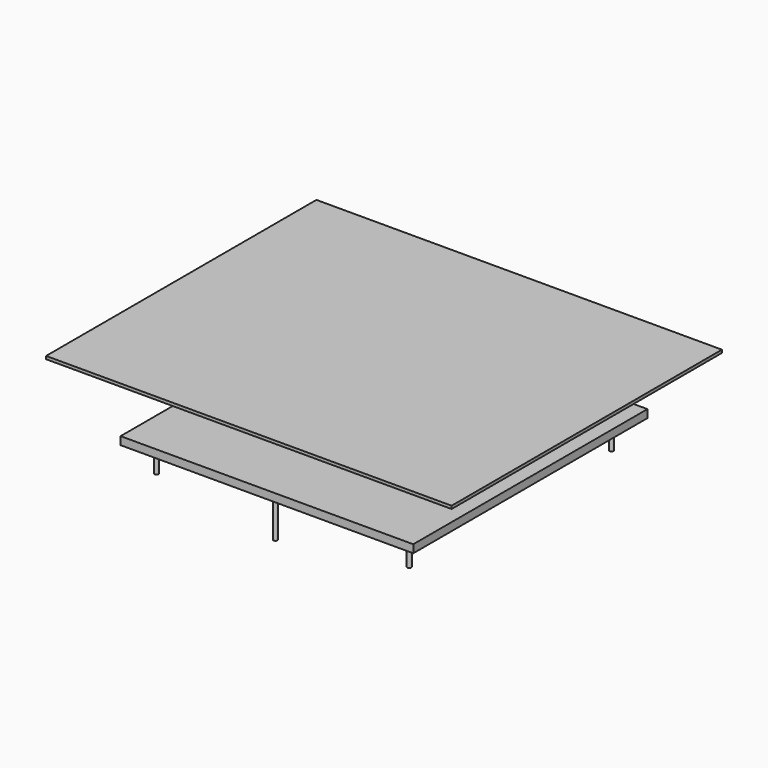
from build123d import *

# Parameters (mm, degrees)
F0_W     = 220
F0_H     = 220
F0_R     = 1.5
F0_W_2   = 200
F0_H_2   = 200
F1_DEPTH = 6
F2_DEPTH = 1.4
F3_DEPTH = 20
F4_DEPTH = 30
F7_W     = 304.8
F7_H     = 254
F8_DEPTH = 2.2


with BuildPart() as f1:
    # F0 (on Top) → F1 (new body)
    with BuildSketch(Plane.XY):
        Rectangle(F0_W, F0_H)
        with Locations((0, -102)):
            Circle(F0_R, mode=Mode.SUBTRACT)
        with Locations((-60, 102)):
            Circle(F0_R, mode=Mode.SUBTRACT)
        Rectangle(F0_W_2, F0_H_2, mode=Mode.SUBTRACT)
        with Locations((60, 102)):
            Circle(F0_R, mode=Mode.SUBTRACT)
        Rectangle(F0_W_2, F0_H_2)
        with Locations((-95, -95)):
            Circle(F0_R, mode=Mode.SUBTRACT)
        with Locations((95, -95)):
            Circle(F0_R, mode=Mode.SUBTRACT)
        with Locations((-95, 95)):
            Circle(F0_R, mode=Mode.SUBTRACT)
        with Locations((95, 95)):
            Circle(F0_R, mode=Mode.SUBTRACT)
        with Locations((-95, 95)):
            Circle(F0_R)
        with Locations((-60, 102)):
            Circle(F0_R)
        with Locations((60, 102)):
            Circle(F0_R)
        with Locations((95, 95)):
            Circle(F0_R)
        with Locations((-95, -95)):
            Circle(F0_R)
        with Locations((0, -102)):
            Circle(F0_R)
        with Locations((95, -95)):
            Circle(F0_R)
    extrude(amount=F1_DEPTH)

    # F0 (on Top) → F2 (join)
    with BuildSketch(Plane.XY):
        Rectangle(F0_W_2, F0_H_2)
        with Locations((-95, -95)):
            Circle(F0_R, mode=Mode.SUBTRACT)
        with Locations((95, -95)):
            Circle(F0_R, mode=Mode.SUBTRACT)
        with Locations((-95, 95)):
            Circle(F0_R, mode=Mode.SUBTRACT)
        with Locations((95, 95)):
            Circle(F0_R, mode=Mode.SUBTRACT)
    extrude(amount=-F2_DEPTH)

    # F0 (on Top) → F3 (join)
    with BuildSketch(Plane.XY):
        with Locations((-95, -95)):
            Circle(F0_R)
        with Locations((95, -95)):
            Circle(F0_R)
        with Locations((-95, 95)):
            Circle(F0_R)
        with Locations((95, 95)):
            Circle(F0_R)
    extrude(amount=-F3_DEPTH)

    # F0 (on Top) → F4 (join)
    with BuildSketch(Plane.XY):
        with Locations((0, -102)):
            Circle(F0_R)
        with Locations((-60, 102)):
            Circle(F0_R)
        with Locations((60, 102)):
            Circle(F0_R)
    extrude(amount=-F4_DEPTH)


with BuildPart() as f8:
    # F7 (on offset) → F8 (new body)
    with BuildSketch(Plane.XY.offset(50)):
        Rectangle(F7_W, F7_H)
    extrude(amount=F8_DEPTH)


solid = Compound([f1.part, f8.part])
